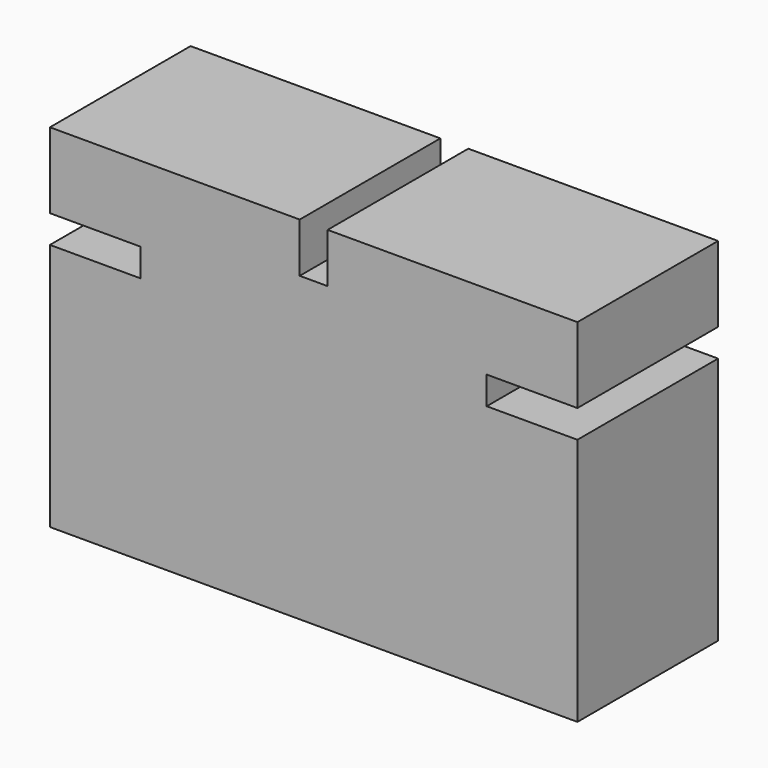
from build123d import *

# Parameters (mm, degrees)
F1_DEPTH = 12.6
F2_R     = 1
F3_DEPTH = 22
F5_DEPTH = 31.301


# Not quite as in the source:
# - a feature names something its author has since deleted; it is built from what else it names


with BuildPart() as f1:
    # F0 (on Front) → F1 (new body)
    with BuildSketch(Plane.XZ):
        Polygon((-1, 12.61), (-18.9, 12.61), (-18.9, 7.19), (-12.4, 7.19), (-12.4, 5.19), (-18.9, 5.19), (-18.9, -12.61), (18.9, -12.61), (18.9, 5.19), (12.4, 5.19), (12.4, 7.19), (18.9, 7.19), (18.9, 12.61), (1, 12.61), (1, 9.06), (0, 9.06), (-1, 9.06), align=None)
    extrude(amount=F1_DEPTH)

    # F2 (on face) → F3 (cut)
    with BuildSketch(Plane(origin=(0, 0, -12.61), x_dir=(1, 0, 0), z_dir=(0, 0, -1))):
        with Locations((0, 6.37)):
            Circle(F2_R)
    extrude(amount=-F3_DEPTH, mode=Mode.SUBTRACT)

    # F4 (on face) → F5 (cut, through all)
    with BuildSketch(Plane(origin=(-12.4, 0, 0), x_dir=(0, -1, 0), z_dir=(-1, 0, 0))):
        with BuildLine():
            ThreePointArc((6.3, 5.19), (7.0071067812, 5.4828932188), (7.3, 6.19))
            ThreePointArc((7.3, 6.19), (7.0071067812, 6.8971067812), (6.3, 7.19))
            ThreePointArc((6.3, 7.19), (5.3, 6.19), (6.3, 5.19))
        make_face()
    extrude(amount=-F5_DEPTH, mode=Mode.SUBTRACT)


solid = f1.part
